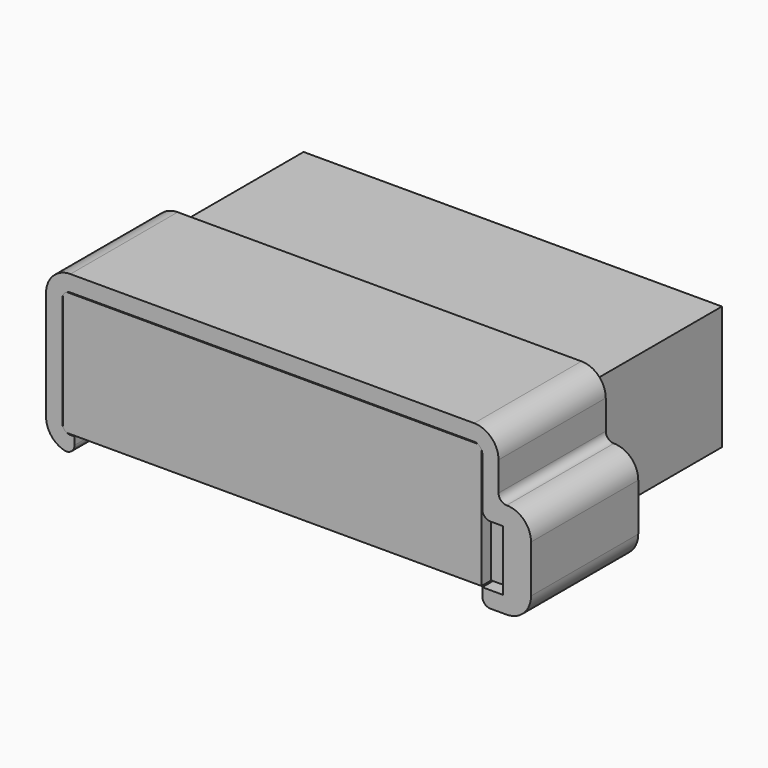
from build123d import *

# Parameters (mm, degrees)
F0_W          = 4
F0_H          = 13.5
F1_DEPTH      = 7.25
F2_DEPTH      = 15.25
F4_START      = 2
F4_DEPTH      = 16.5
F6_DEPTH      = 0.1
F6_DEPTH_BACK = 7.35
F7_R          = 0.99999


# Not quite as in the source:
# - a fillet or chamfer is up to 0.001 mm smaller than in the source, because OpenCascade refuses the exact size


with BuildPart() as f1:
    # F0 (on Top) → F1 (new body)
    with BuildSketch(Plane.XY):
        with Locations((27.75, -10.25)):
            Rectangle(F0_W, F0_H)
    extrude(amount=F1_DEPTH)

    # F0 (on Top) → F2 (join)
    with BuildSketch(Plane.XY):
        Polygon((25.75, 18.5), (-25.75, 18.5), (-25.75, -18.5), (25.75, -18.5), (25.75, -17), (25.75, -3.5), align=None)
    extrude(amount=F2_DEPTH)


with BuildPart() as f4:
    # F3 (on Front) → F4 (new body)
    with BuildSketch(Plane.XZ.offset(F4_START)):
        with BuildLine():
            Line((-24.85, 15.35), (24.85, 15.35))
            ThreePointArc((24.85, 15.35), (25.5571067812, 15.0571067812), (25.85, 14.35))
            Line((25.85, 14.35), (25.85, 7.35))
            Line((25.85, 7.35), (28.85, 7.35))
            ThreePointArc((28.85, 7.35), (29.5571067812, 7.0571067812), (29.85, 6.35))
            Line((29.85, 6.35), (29.85, 0.9))
            ThreePointArc((29.85, 0.9), (29.5571067812, 0.1928932188), (28.85, -0.1))
            Line((28.85, -0.1), (26, -0.1))
            Line((26, -0.1), (25.85, -0.1))
            Line((25.85, -0.1), (25.85, -2.1))
            Line((25.85, -2.1), (26, -2.1))
            Line((26, -2.1), (28.85, -2.1))
            ThreePointArc((28.85, -2.1), (30.9713203436, -1.2213203436), (31.85, 0.9))
            Line((31.85, 0.9), (31.85, 6.75))
            ThreePointArc((31.85, 6.75), (30.9713203436, 8.8713203436), (28.85, 9.75))
            Line((28.85, 9.75), (27.85, 9.75))
            Line((27.85, 9.75), (27.85, 14.35))
            ThreePointArc((27.85, 14.35), (26.9713203436, 16.4713203436), (24.85, 17.35))
            Line((24.85, 17.35), (-24.85, 17.35))
            ThreePointArc((-24.85, 17.35), (-26.9713203436, 16.4713203436), (-27.85, 14.35))
            Line((-27.85, 14.35), (-27.85, 0.9))
            ThreePointArc((-27.85, 0.9), (-26.9713203436, -1.2213203436), (-24.85, -2.1))
            Line((-24.85, -2.1), (-24.35, -2.1))
            Line((-24.35, -2.1), (-24.35, -0.1))
            Line((-24.35, -0.1), (-24.85, -0.1))
            ThreePointArc((-24.85, -0.1), (-25.5571067812, 0.1928932188), (-25.85, 0.9))
            Line((-25.85, 0.9), (-25.85, 14.35))
            ThreePointArc((-25.85, 14.35), (-25.5571067812, 15.0571067812), (-24.85, 15.35))
        make_face()
    extrude(amount=F4_DEPTH)

    # F5 (on Top) → F6 (join, two sides)
    with BuildSketch(Plane.XY) as f6_sk:
        Polygon((29.85, -3.4585786438), (29.85, -2.0000000002), (28.3914213564, -2.0000000001), align=None)
        Polygon((28.3914213559, -18.5000000004), (29.85, -18.5000000004), (29.85, -17.0414213562), align=None)
    extrude(amount=-F6_DEPTH)
    extrude(f6_sk.sketch, amount=F6_DEPTH_BACK)

    # F7 (radius 1 in the source; OpenCascade refuses exactly that, so slightly less here)
    f7_edges = [f4.edges().sort_by_distance(p)[0] for p in [
        (25.85, -10.25, 7.35),
        (27.85, -10.25, 9.75),
        (-24.35, -10.25, -2.1),
        (25.85, -10.25, -2.1),
    ]]
    fillet(f7_edges, radius=F7_R)


solid = Compound([f1.part, f4.part])
